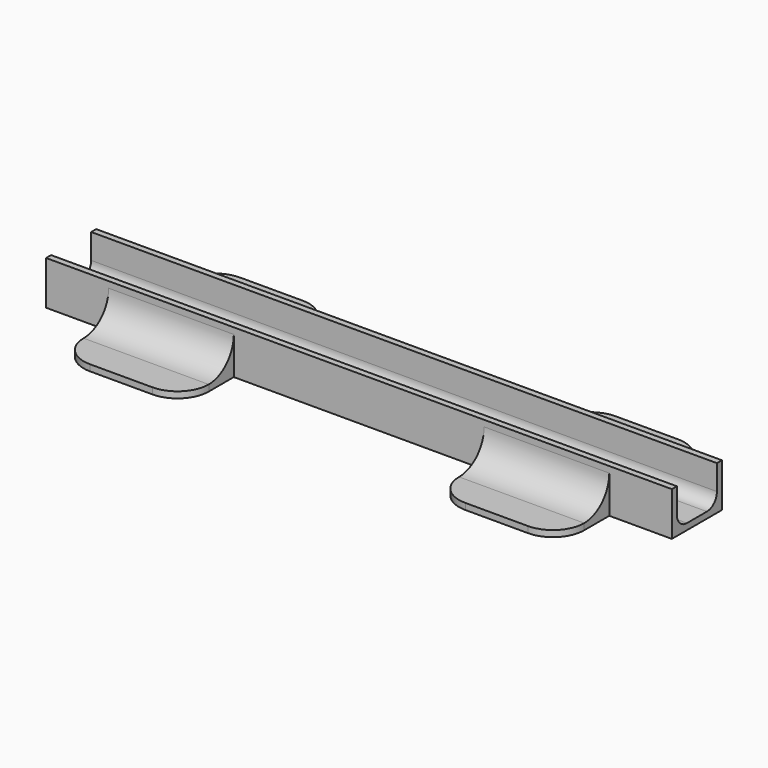
from build123d import *

# Parameters (mm, degrees)
F1_DEPTH = 100
F2_W     = 20
F2_H     = 30
F3_DEPTH = 1
F4_R     = 4.99999
F5_R     = 2


# Not quite as in the source:
# - a fillet or chamfer is up to 0.001 mm smaller than in the source, because OpenCascade refuses the exact size


with BuildPart() as f1:
    # F0 (on Right) → F1 (new body)
    with BuildSketch(Plane.YZ):
        Polygon((-4, 7), (-5, 7), (-5, 0), (5, 0), (5, 7), (4, 7), (4, 1), (-4, 1), align=None)
    extrude(amount=F1_DEPTH)

    # F2 (on Top) → F3 (join)
    with BuildSketch(Plane.XY):
        with Locations((20, 0)):
            Rectangle(F2_W, F2_H)
        with Locations((80, 0)):
            Rectangle(F2_W, F2_H)
    extrude(amount=F3_DEPTH)

    # F4 (radius 5 in the source; OpenCascade refuses exactly that, so slightly less here)
    f4_edges = [f1.edges().sort_by_distance(p)[0] for p in [
        (20, -5, 1),
        (80, -5, 1),
        (20, 5, 1),
        (80, 5, 1),
        (10, -15, 0.5),
        (30, -15, 0.5),
        (70, -15, 0.5),
        (90, -15, 0.5),
        (10, 15, 0.5),
        (30, 15, 0.5),
        (70, 15, 0.5),
        (90, 15, 0.5),
    ]]
    fillet(f4_edges, radius=F4_R)

    # F5
    f5_edges = [f1.edges().sort_by_distance(p)[0] for p in [
        (50, 4, 1),
        (50, -4, 1),
    ]]
    fillet(f5_edges, radius=F5_R)


solid = f1.part
